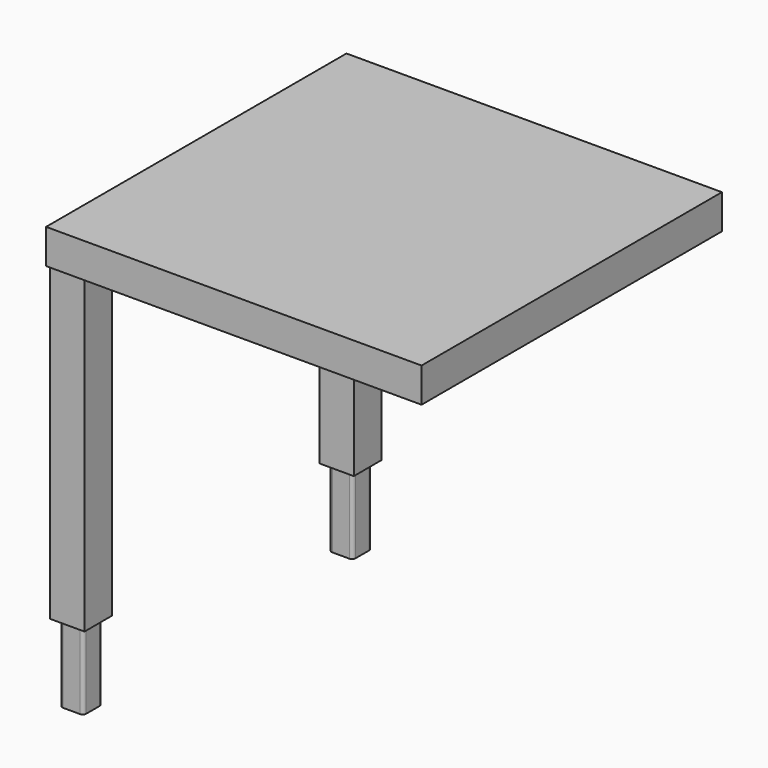
from build123d import *

# Parameters (mm, degrees)
F1_W      = 50.8
F1_H      = 50.8
F2_DEPTH  = 508
F5_W      = 50.8
F5_H      = 50.8
F6_DEPTH  = 50.8
F8_W      = 552.45
F8_H      = 552.45
F8_W_2    = 546.1
F8_H_2    = 546.1
F9_DEPTH  = 50.8
F10_DEPTH = 457.2
F12_DEPTH = 114.3
F13_R     = 5.08


# Not quite as in the source:
# - a pattern or mirror of a feature is missing from the dataset's text; its kind, count and spacing are read off the source's solid


with BuildPart() as f2:
    # F1 (on Top) → F2 (new body)
    with BuildSketch(Plane.XY):
        with Locations((-247.65, 247.65)):
            Rectangle(F1_W, F1_H)
    extrude(amount=F2_DEPTH)


with BuildPart() as f3_1:
    # F3: instance of F2
    add(f2.part.mirror(Plane.YZ))


with BuildPart() as f4_1:
    # F4: instance of F2
    add(f2.part.mirror(Plane.XZ))


with BuildPart() as f4_2:
    # F4: instance of F3_1
    add(f3_1.part.mirror(Plane.XZ))


with BuildPart() as f2_1:
    add(f2.part)

    add(f3_1.part)  # F6 merges F3_1

    add(f4_1.part)  # F6 merges F4_1

    add(f4_2.part)  # F6 merges F4_2
    # F5 (on face) → F6 (join)
    with BuildSketch(Plane.XY.offset(508)):
        Polygon((-273.05, 222.25), (-273.05, -273.05), (273.05, -273.05), (273.05, 273.05), (-222.25, 273.05), (-222.25, 222.25), align=None)
        with Locations((-247.65, 247.65)):
            Rectangle(F5_W, F5_H)
    extrude(amount=-F6_DEPTH)

    # F7: union 

    # F8 (on face) → F9 (join, through all)
    with BuildSketch(Plane.XY.offset(508)):
        Rectangle(F8_W, F8_H)
        Rectangle(F8_W_2, F8_H_2, mode=Mode.SUBTRACT)
    extrude(amount=-F9_DEPTH)

    # F10 (cut, through all): faces of the model
    f10_faces = [f2_1.faces().sort_by_distance(p)[0] for p in [
        (247.65, -247.65, 0),
        (247.65, 247.65, 0),
    ]]
    extrude(f10_faces, amount=-F10_DEPTH, mode=Mode.SUBTRACT)

    # F11 (on face) → F12 (join)
    with BuildSketch(Plane(origin=(0, 0, 0), x_dir=(1, 0, 0), z_dir=(0, 0, -1))):
        Polygon((-230.124, 265.176), (-265.176, 265.176), (-230.124, 230.124), align=None)
        Polygon((-230.124, 230.124), (-265.176, 265.176), (-265.176, 230.124), align=None)
    f12 = extrude(amount=F12_DEPTH)

    # F12_copies: F12 across plane
    add(f12.mirror(Plane.ZX))

    # F13
    f13_edges = [f2_1.edges().sort_by_distance(p)[0] for p in [
        (-230.124, -265.176, -57.15),
        (-265.176, -265.176, -57.15),
        (-230.124, -230.124, -57.15),
        (-265.176, -230.124, -57.15),
        (-230.124, 265.176, -57.15),
        (-265.176, 265.176, -57.15),
        (-265.176, 230.124, -57.15),
        (-230.124, 230.124, -57.15),
    ]]
    fillet(f13_edges, radius=F13_R)


solid = f2_1.part
